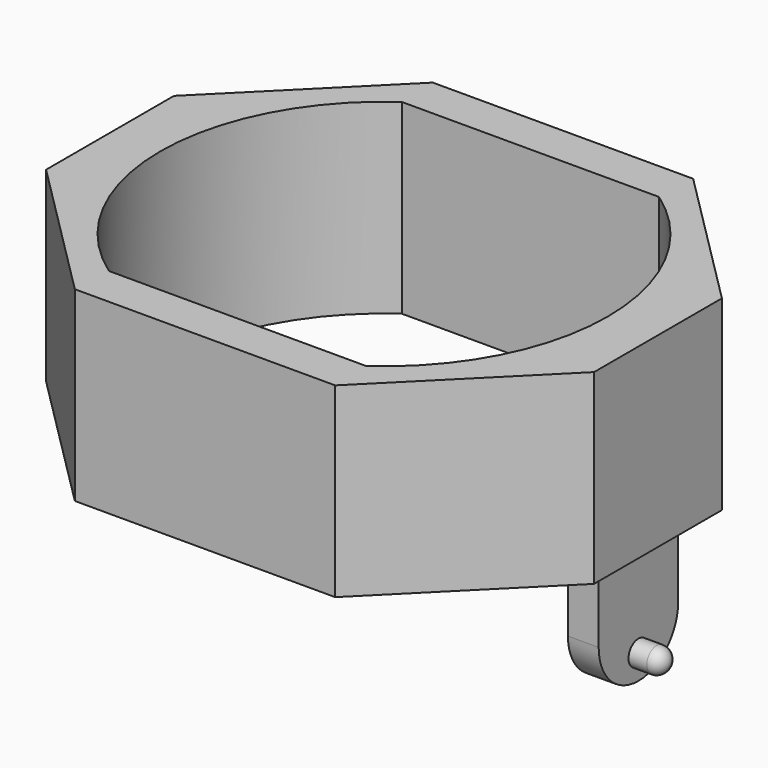
from build123d import *

# Parameters (mm, degrees)
F1_DEPTH  = 19.05
F3_DEPTH  = 6.35
F4_R      = 0.635
F5_DEPTH  = 1.5691231
F6_R      = 2.53999
F7_R      = 0.635
F9_DEPTH  = 6.35
F11_D     = 2.54
F16_D     = 127
F16_DEPTH = 15.876


# Not quite as in the source:
# - a fillet or chamfer is up to 0.001 mm smaller than in the source, because OpenCascade refuses the exact size
# - a length typed as a fraction of an inch, garbled in the dataset ("3 / 203.2 mm" for 3/8 in), is restored
# - the program builds the solid bodies; features that only make, move or delete a surface that nothing else refers to are left out


with BuildPart() as f1:
    # F0 (on Top) → F1 (new body)
    with BuildSketch(Plane.XY):
        Polygon((6.6501818182, 11.43), (0, 11.43), (-6.6501818182, 11.43), (-13.9976640991, 4.0825177191), (-13.9976640991, 0), (-13.9976640991, -4.0825177191), (-6.6501818182, -11.43), (0, -11.43), (6.6501818182, -11.43), (13.9976640991, -4.0825177191), (13.9976640991, 0), (13.9976640991, 4.0825177191), align=None)
        with BuildLine():
            ThreePointArc((6.5717879374, 9.3518181818), (10.1429886159, 5.26922024), (11.43, 0))
            ThreePointArc((11.43, 0), (10.1429886159, -5.26922024), (6.5717879374, -9.3518181818))
            Line((6.5717879374, -9.3518181818), (0, -9.3518181818))
            Line((0, -9.3518181818), (-6.5717879374, -9.3518181818))
            ThreePointArc((-6.5717879374, -9.3518181818), (-10.1429886159, -5.26922024), (-11.43, 0))
            ThreePointArc((-11.43, 0), (-10.1429886159, 5.26922024), (-6.5717879374, 9.3518181818))
            Line((-6.5717879374, 9.3518181818), (0, 9.3518181818))
            Line((0, 9.3518181818), (6.5717879374, 9.3518181818))
        make_face(mode=Mode.SUBTRACT)
    extrude(amount=F1_DEPTH)

    # F2 (on Top) → F3 (join)
    with BuildSketch(Plane.XY):
        Polygon((12.9991231, -2.54), (12.9991231, 0), (12.9991231, 2.54), (11.43, 2.54), (11.43, 0), (11.43, -2.54), align=None)
    extrude(amount=-F3_DEPTH)

    # F4 (on face) → F5 (join)
    with BuildSketch(Plane.YZ.offset(12.9991231)):
        with Locations((0, -5.08)):
            Circle(F4_R)
    extrude(amount=F5_DEPTH)

    # F6 (radius 2.54 in the source; OpenCascade refuses exactly that, so slightly less here)
    f6_edges = [f1.edges().sort_by_distance(p)[0] for p in [
        (12.214562, -2.54, -6.35),
        (12.214562, 2.54, -6.35),
    ]]
    fillet(f6_edges, radius=F6_R)

    # F7
    f7_edges = [f1.edges().sort_by_distance(p)[0] for p in [
        (14.568246, -0.635, -5.08),
    ]]
    fillet(f7_edges, radius=F7_R)

    # F8 (on face) → F9 (join)
    with BuildSketch(Plane.XY.offset(19.05)):
        Polygon((13.9976640991, 2.54), (12.4285360385, 2.54), (12.4285360385, 0), (12.4285360385, -2.54), (13.9976640991, -2.54), (13.9976640991, 0), align=None)
    extrude(amount=F9_DEPTH)

    # F11 (through all)
    with Locations(Plane.YZ.offset(13.9976640991)):
        with Locations((0, 22.86)):
            Hole(F11_D / 2)

    # F12: F1 across plane


with BuildPart() as f1_1:
    add(f1.part)
    add(f1.part.mirror(Plane.YZ))

    # F16 (through all, one way)
    with BuildSketch(Plane(origin=(0, 0, 9.525), x_dir=(1, 0, 0), z_dir=(0, 0, -1))):
        with Locations((0, 0)):
            Circle(F16_D / 2)
    extrude(amount=-F16_DEPTH, mode=Mode.SUBTRACT)


solid = f1_1.part
